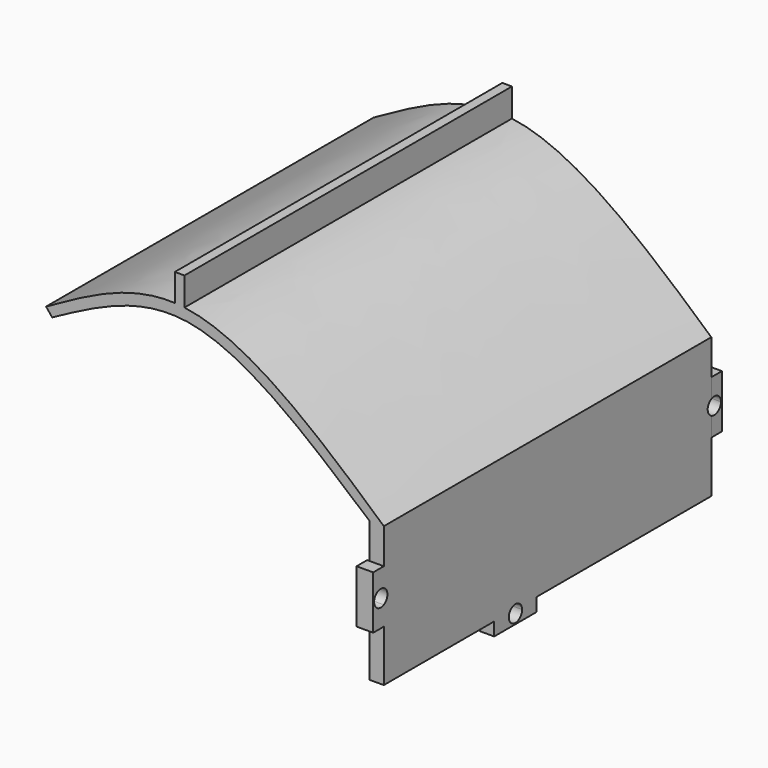
from build123d import *
from build123d import SkipClean  # not in build123d's __all__

# Parameters (mm, degrees)
F0_W     = 3.048
F0_H     = 29.9492416
F1_DEPTH = 87.63
F2_R     = 1.778
F3_DEPTH = 3.048
F4_DEPTH = 25.4
F5_DEPTH = 25.4
F6_DEPTH = 3.556
F7_DEPTH = 3.556


with BuildPart() as f1:
    # F0 (on Front) → F1 (new body)
    with BuildSketch(Plane.XZ):
        with BuildLine():
            add(Edge.make_bspline(
                [(-69.252148823, 47.2862608473), (-60.3127224637, 52.3166042602), (-51.4062820573, 57.4050875064), (-41.6824767012, 56.9220757762)],
                knots=[0, 0, 0, 0, 0.4104821983, 0.4104821983, 0.4104821983, 0.4104821983], degree=3))
            Line((-69.252148823, 47.2862608473), (-67.9539144039, 45.6614680588))
            add(Edge.make_bspline(
                [(0, 29.4084157124), (-13.5805348603, 41.0502040776), (-37.9650308205, 61.9535885379), (-58.746385608, 50.6636605559), (-67.9539144039, 45.6614680588)],
                knots=[0, 0, 0, 0, 0.5569331793, 1, 1, 1, 1], degree=3))
            Line((0, 29.4084157124), (3.048, 29.4084157124))
            add(Edge.make_bspline(
                [(-39.6240018308, 56.7362643778), (-26.1787631346, 54.9709717695), (-11.0970199105, 42.072411724), (3.048, 29.4084157124)],
                knots=[0.4392739055, 0.4392739055, 0.4392739055, 0.4392739055, 1, 1, 1, 1], degree=3))
            add(Edge.make_bspline(
                [(-41.6824767012, 56.9220757762), (-41.0004374843, 56.8881967617), (-40.3143770071, 56.8269071863), (-39.6240018308, 56.7362643778)],
                knots=[0.4104821983, 0.4104821983, 0.4104821983, 0.4104821983, 0.4392739055, 0.4392739055, 0.4392739055, 0.4392739055], degree=3))
        make_face()
        with BuildLine():
            Line((-41.6824767012, 62.7852019621), (-41.6824767012, 56.9220757762))
            add(Edge.make_bspline(
                [(-41.6824767012, 56.9220757762), (-41.0004374843, 56.8881967617), (-40.3143770071, 56.8269071863), (-39.6240018308, 56.7362643778)],
                knots=[0.4104821983, 0.4104821983, 0.4104821983, 0.4104821983, 0.4392739055, 0.4392739055, 0.4392739055, 0.4392739055], degree=3))
            Line((-39.6240018308, 56.7362643778), (-39.6240018308, 62.7852019621))
            Line((-39.6240018308, 62.7852019621), (-41.6824767012, 62.7852019621))
        make_face()
        with Locations((1.524, 14.4337949124)):
            Rectangle(F0_W, F0_H)
    extrude(amount=F1_DEPTH)

    # F2 (on face) → F3 (join)
    with BuildSketch(Plane.YZ.offset(3.048)):
        with Locations((-52.4002, -1.3536258876)):
            Circle(F2_R)
        with Locations((-88.4428, 16.1723741124)):
            Circle(F2_R)
        with Locations((0.8128, 16.1723741124)):
            Circle(F2_R)
        with BuildLine():
            Line((-53.9815412535, -0.5408258876), (-58.0898, -0.5408258876))
            Line((-58.0898, -0.5408258876), (-58.0898, -3.3856258876))
            Line((-58.0898, -3.3856258876), (-46.7106, -3.3856258876))
            Line((-46.7106, -3.3856258876), (-46.7106, -0.5408258876))
            Line((-46.7106, -0.5408258876), (-50.8188587465, -0.5408258876))
            ThreePointArc((-50.8188587465, -0.5408258876), (-50.6720639017, -0.9354995602), (-50.6222, -1.3536258876))
            ThreePointArc((-50.6222, -1.3536258876), (-52.8183263274, -3.0817619859), (-53.9815412535, -0.5408258876))
        make_face()
    extrude(amount=-F3_DEPTH)

    # F2 (on face) → F4 (cut)
    with BuildSketch(Plane.YZ.offset(3.048)):
        with BuildLine():
            ThreePointArc((-50.8188587465, -0.5408258876), (-52.4002, 0.4243741124), (-53.9815412535, -0.5408258876))
            Line((-53.9815412535, -0.5408258876), (-50.8188587465, -0.5408258876))
        make_face()
        with BuildLine():
            Line((-50.8188587465, -0.5408258876), (-53.9815412535, -0.5408258876))
            ThreePointArc((-53.9815412535, -0.5408258876), (-52.8183263274, -3.0817619859), (-50.6222, -1.3536258876))
            ThreePointArc((-50.6222, -1.3536258876), (-50.6720639017, -0.9354995602), (-50.8188587465, -0.5408258876))
        make_face()
    extrude(amount=-F4_DEPTH, mode=Mode.SUBTRACT)

    # F2 (on face) → F5 (cut)
    with BuildSketch(Plane.YZ.offset(3.048)):
        with Locations((-52.4002, -1.3536258876)):
            Circle(F2_R)
        with Locations((-88.4428, 16.1723741124)):
            Circle(F2_R)
        with Locations((0.8128, 16.1723741124)):
            Circle(F2_R)
        with BuildLine():
            Line((-87.63, 17.7537153659), (-87.63, 14.5910328589))
            ThreePointArc((-87.63, 14.5910328589), (-86.9251632846, 15.24605732), (-86.6648, 16.1723741124))
            ThreePointArc((-86.6648, 16.1723741124), (-86.9251632846, 17.0986909049), (-87.63, 17.7537153659))
        make_face()
    extrude(amount=-F5_DEPTH, mode=Mode.SUBTRACT)

    # F2 (on face) → F6 (join)
    with BuildSketch(Plane.YZ.offset(3.048)):
        with BuildLine():
            Line((-90.4748, 10.4827741124), (-87.63, 10.4827741124))
            Line((-87.63, 10.4827741124), (-87.63, 14.5910328589))
            ThreePointArc((-87.63, 14.5910328589), (-90.2208, 16.1723741124), (-87.63, 17.7537153659))
            Line((-87.63, 17.7537153659), (-87.63, 21.8619741124))
            Line((-87.63, 21.8619741124), (-90.4748, 21.8619741124))
            Line((-90.4748, 21.8619741124), (-90.4748, 10.4827741124))
        make_face()
    extrude(amount=-F6_DEPTH)

    # F2 (on face) → F7 (join)
    with BuildSketch(Plane.YZ.offset(3.048)):
        with BuildLine():
            Line((0, 14.5910328589), (0, 10.4827741124))
            Line((0, 10.4827741124), (2.8448, 10.4827741124))
            Line((2.8448, 10.4827741124), (2.8448, 21.8619741124))
            Line((2.8448, 21.8619741124), (0, 21.8619741124))
            Line((0, 21.8619741124), (0, 17.7537153659))
            ThreePointArc((0, 17.7537153659), (1.7391167925, 17.6900108278), (2.5908, 16.1723741124))
            ThreePointArc((2.5908, 16.1723741124), (1.7391167925, 14.654737397), (0, 14.5910328589))
        make_face()
    with SkipClean():  # cleaning this boolean's faces spoils the solid; the shape is the same uncleaned
        extrude(amount=-F7_DEPTH)


solid = f1.part
